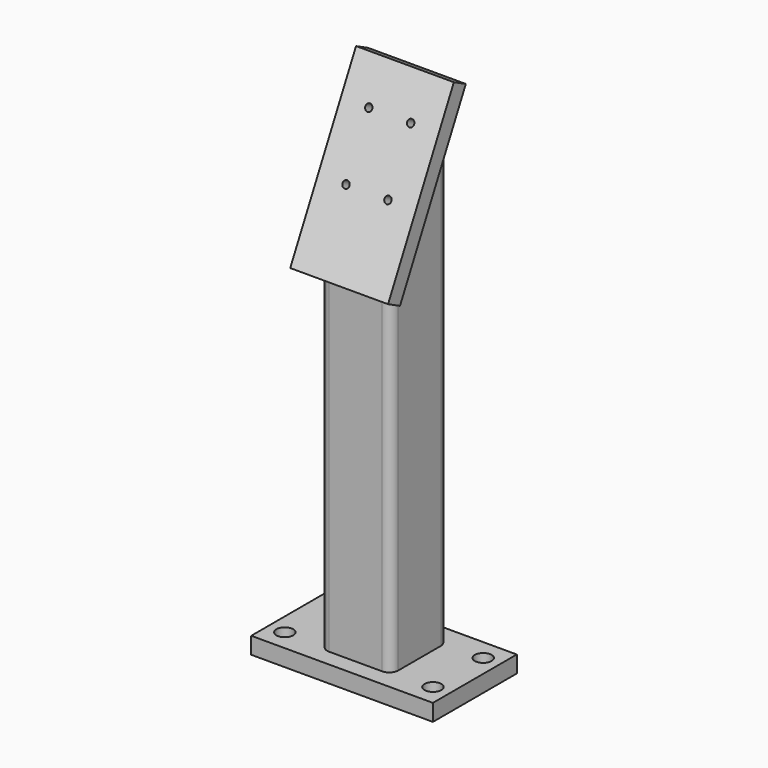
from build123d import *

# Parameters (mm, degrees)
F0_W      = 130
F0_H      = 75
F1_DEPTH  = 12
F3_DEPTH  = 345
F5_D      = 12
F7_DEPTH  = 50.8
F8_W      = 70
F8_H      = 130
F9_DEPTH  = 12
F11_D     = 5
F11_DEPTH = 8
F11_TIP   = 1.5021515476


with BuildPart() as f1:
    # F0 (on Top) → F1 (new body)
    with BuildSketch(Plane.XY):
        Rectangle(F0_W, F0_H)
    extrude(amount=-F1_DEPTH)

    # F2 (on face) → F3 (join)
    with BuildSketch(Plane.XY):
        with BuildLine():
            Line((-19.05, -25.4), (19.05, -25.4))
            ThreePointArc((19.05, -25.4), (23.5401280605, -23.5401280605), (25.4, -19.05))
            Line((25.4, -19.05), (25.4, 19.05))
            ThreePointArc((25.4, 19.05), (23.5401280605, 23.5401280605), (19.05, 25.4))
            Line((19.05, 25.4), (-19.05, 25.4))
            ThreePointArc((-19.05, 25.4), (-23.5401280605, 23.5401280605), (-25.4, 19.05))
            Line((-25.4, 19.05), (-25.4, -19.05))
            ThreePointArc((-25.4, -19.05), (-23.5401280605, -23.5401280605), (-19.05, -25.4))
        make_face()
        with BuildLine():
            Line((-12.7, 19.05), (12.7, 19.05))
            ThreePointArc((12.7, 19.05), (17.1901280605, 17.1901280605), (19.05, 12.7))
            Line((19.05, 12.7), (19.05, -12.7))
            ThreePointArc((19.05, -12.7), (17.1901280605, -17.1901280605), (12.7, -19.05))
            Line((12.7, -19.05), (-12.7, -19.05))
            ThreePointArc((-12.7, -19.05), (-17.1901280605, -17.1901280605), (-19.05, -12.7))
            Line((-19.05, -12.7), (-19.05, 12.7))
            ThreePointArc((-19.05, 12.7), (-17.1901280605, 17.1901280605), (-12.7, 19.05))
        make_face(mode=Mode.SUBTRACT)
    extrude(amount=F3_DEPTH)

    # F5 (through all)
    with Locations(Plane.XY):
        with Locations((-53, 22.5), (53, 22.5), (53, -22.5), (-53, -22.5)):
            Hole(F5_D / 2)

    # F6 (on face) → F7 (cut)
    with BuildSketch(Plane.YZ.offset(25.4)):
        Polygon((-19.05, 345), (-25.4, 345), (-25.4, 244.9542985566), (-19.05, 257.460011237), align=None)
        Polygon((19.05, 345), (-19.05, 345), (-19.05, 257.460011237), (19.05, 332.4942873196), align=None)
        Polygon((25.4, 345), (19.05, 345), (19.05, 332.4942873196), align=None)
    extrude(amount=-F7_DEPTH, mode=Mode.SUBTRACT)

    # F8 (on face) → F9 (join)
    with BuildSketch(Plane(origin=(0, -119.0782097883, 60.4640976071), x_dir=(1, 0, 0), z_dir=(0, -0.8916395458, 0.4527459778))):
        with Locations((0, 263.0132913952)):
            Rectangle(F8_W, F8_H)
        with BuildLine():
            Line((25.4, 305.0898661941), (25.4, 220.9367165963))
            add(Edge.make_bspline(
                [(25.4, 220.9367165963), (25.4, 206.9111916633), (19.05, 206.9111916633)],
                knots=[4.7123889804, 4.7123889804, 4.7123889804, 6.2831853072, 6.2831853072, 6.2831853072], degree=2, weights=[1, 0.7071067812, 1]))
            Line((19.05, 206.9111916633), (-19.05, 206.9111916633))
            add(Edge.make_bspline(
                [(-19.05, 206.9111916633), (-25.4, 206.9111916633), (-25.4, 220.9367165963)],
                knots=[0, 0, 0, 1.5707963268, 1.5707963268, 1.5707963268], degree=2, weights=[1, 0.7071067812, 1]))
            Line((-25.4, 220.9367165963), (-25.4, 305.0898661941))
            add(Edge.make_bspline(
                [(-25.4, 305.0898661941), (-25.4, 319.115391127), (-19.05, 319.115391127)],
                knots=[1.5707963268, 1.5707963268, 1.5707963268, 3.1415926536, 3.1415926536, 3.1415926536], degree=2, weights=[1, 0.7071067812, 1]))
            Line((-19.05, 319.115391127), (19.05, 319.115391127))
            add(Edge.make_bspline(
                [(19.05, 319.115391127), (25.4, 319.115391127), (25.4, 305.0898661941)],
                knots=[3.1415926536, 3.1415926536, 3.1415926536, 4.7123889804, 4.7123889804, 4.7123889804], degree=2, weights=[1, 0.7071067812, 1]))
        make_face(mode=Mode.SUBTRACT)
        with BuildLine():
            add(Edge.make_bspline(
                [(25.4, 220.9367165963), (25.4, 206.9111916633), (19.05, 206.9111916633)],
                knots=[4.7123889804, 4.7123889804, 4.7123889804, 6.2831853072, 6.2831853072, 6.2831853072], degree=2, weights=[1, 0.7071067812, 1]))
            Line((25.4, 220.9367165963), (25.4, 305.0898661941))
            add(Edge.make_bspline(
                [(19.05, 319.115391127), (25.4, 319.115391127), (25.4, 305.0898661941)],
                knots=[3.1415926536, 3.1415926536, 3.1415926536, 4.7123889804, 4.7123889804, 4.7123889804], degree=2, weights=[1, 0.7071067812, 1]))
            Line((19.05, 319.115391127), (-19.05, 319.115391127))
            add(Edge.make_bspline(
                [(-25.4, 305.0898661941), (-25.4, 319.115391127), (-19.05, 319.115391127)],
                knots=[1.5707963268, 1.5707963268, 1.5707963268, 3.1415926536, 3.1415926536, 3.1415926536], degree=2, weights=[1, 0.7071067812, 1]))
            Line((-25.4, 305.0898661941), (-25.4, 220.9367165963))
            add(Edge.make_bspline(
                [(-19.05, 206.9111916633), (-25.4, 206.9111916633), (-25.4, 220.9367165963)],
                knots=[0, 0, 0, 1.5707963268, 1.5707963268, 1.5707963268], degree=2, weights=[1, 0.7071067812, 1]))
            Line((-19.05, 206.9111916633), (19.05, 206.9111916633))
        make_face()
        with BuildLine():
            Line((-19.05, 234.9622415292), (-19.05, 291.0643412611))
            add(Edge.make_bspline(
                [(-19.05, 291.0643412611), (-19.05, 305.0898661941), (-12.7, 305.0898661941)],
                knots=[1.5707963268, 1.5707963268, 1.5707963268, 3.1415926536, 3.1415926536, 3.1415926536], degree=2, weights=[1, 0.7071067812, 1]))
            Line((-12.7, 305.0898661941), (12.7, 305.0898661941))
            add(Edge.make_bspline(
                [(12.7, 305.0898661941), (19.05, 305.0898661941), (19.05, 291.0643412611)],
                knots=[3.1415926536, 3.1415926536, 3.1415926536, 4.7123889804, 4.7123889804, 4.7123889804], degree=2, weights=[1, 0.7071067812, 1]))
            Line((19.05, 291.0643412611), (19.05, 234.9622415292))
            add(Edge.make_bspline(
                [(19.05, 234.9622415292), (19.05, 220.9367165963), (12.7, 220.9367165963)],
                knots=[4.7123889804, 4.7123889804, 4.7123889804, 6.2831853072, 6.2831853072, 6.2831853072], degree=2, weights=[1, 0.7071067812, 1]))
            Line((12.7, 220.9367165963), (-12.7, 220.9367165963))
            add(Edge.make_bspline(
                [(-12.7, 220.9367165963), (-19.05, 220.9367165963), (-19.05, 234.9622415292)],
                knots=[0, 0, 0, 1.5707963268, 1.5707963268, 1.5707963268], degree=2, weights=[1, 0.7071067812, 1]))
        make_face(mode=Mode.SUBTRACT)
        with BuildLine():
            add(Edge.make_bspline(
                [(-19.05, 291.0643412611), (-19.05, 305.0898661941), (-12.7, 305.0898661941)],
                knots=[1.5707963268, 1.5707963268, 1.5707963268, 3.1415926536, 3.1415926536, 3.1415926536], degree=2, weights=[1, 0.7071067812, 1]))
            Line((-19.05, 291.0643412611), (-19.05, 234.9622415292))
            add(Edge.make_bspline(
                [(-12.7, 220.9367165963), (-19.05, 220.9367165963), (-19.05, 234.9622415292)],
                knots=[0, 0, 0, 1.5707963268, 1.5707963268, 1.5707963268], degree=2, weights=[1, 0.7071067812, 1]))
            Line((-12.7, 220.9367165963), (12.7, 220.9367165963))
            add(Edge.make_bspline(
                [(19.05, 234.9622415292), (19.05, 220.9367165963), (12.7, 220.9367165963)],
                knots=[4.7123889804, 4.7123889804, 4.7123889804, 6.2831853072, 6.2831853072, 6.2831853072], degree=2, weights=[1, 0.7071067812, 1]))
            Line((19.05, 234.9622415292), (19.05, 291.0643412611))
            add(Edge.make_bspline(
                [(12.7, 305.0898661941), (19.05, 305.0898661941), (19.05, 291.0643412611)],
                knots=[3.1415926536, 3.1415926536, 3.1415926536, 4.7123889804, 4.7123889804, 4.7123889804], degree=2, weights=[1, 0.7071067812, 1]))
            Line((12.7, 305.0898661941), (-12.7, 305.0898661941))
        make_face()
    extrude(amount=F9_DEPTH)

    # F11
    with Locations(Plane(origin=(0, -129.7778843376, 65.8970493408), x_dir=(1, 0, 0), z_dir=(0, -0.8916395458, 0.4527459778))):
        with Locations((15, 298.0132913952), (15, 253.0132913952), (-15, 253.0132913952), (-15, 298.0132913952)):
            Hole(F11_D / 2, depth=F11_DEPTH)
            with Locations((0, 0, -(F11_DEPTH + F11_TIP / 2))):  # 118° drill point
                Cone(0, F11_D / 2, F11_TIP, mode=Mode.SUBTRACT)


solid = f1.part
